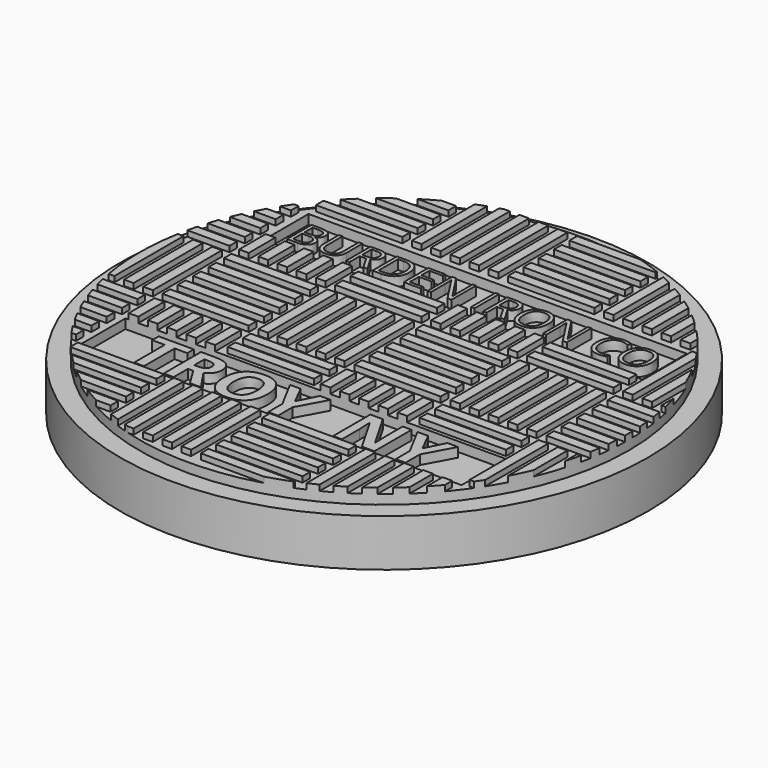
from build123d import *

# Parameters (mm, degrees)
F0_R           = 27.94
F1_DEPTH       = 6
F2_W           = 1.016
F2_H           = 9.144
F2_W_2         = 9.144
F2_H_2         = 1.016
F3_DEPTH       = 0.6
F4_R           = 47.3051944378
F4_R_2         = 27.94
F5_DEPTH       = 25.4
F6_DEPTH       = 5
F7_R           = 27.94
F7_R_2         = 25.908
F8_DEPTH       = 25.4
F9_W           = 40.0505103171
F9_H           = 5.9277797118
F10_DEPTH      = 25.4
F11_TEXT_SIZE  = 4.5379089589
F12_DEPTH      = 1
F12_DEPTH_BACK = 1
F13_W          = 40.3386186808
F13_H          = 5.9581985697
F14_DEPTH      = 25.4
F15_TEXT_SIZE  = 6.8953818821
F16_DEPTH      = 1


# Not quite as in the source:
# - Text() gives the source's letters only with a copy of the font that has no kerning and outlines rounded to 1/6400 em; it was checked with that copy


with BuildPart() as f1:
    # F0 (on Top) → F1 (new body)
    with BuildSketch(Plane.XY):
        Circle(F0_R)
    extrude(amount=F1_DEPTH)

    # F2 (on face) → F3 (join)
    with BuildSketch(Plane.XY.offset(6)):
        with Locations((-9.144, 0)):
            Rectangle(F2_W, F2_H)
        with Locations((-7.112, 0)):
            Rectangle(F2_W, F2_H)
        with Locations((-5.08, 0)):
            Rectangle(F2_W, F2_H)
        with Locations((-3.048, 0)):
            Rectangle(F2_W, F2_H)
        with Locations((-1.016, 0)):
            Rectangle(F2_W, F2_H)
        with Locations((5.08, 4.064)):
            Rectangle(F2_W_2, F2_H_2)
        with Locations((5.08, 2.032)):
            Rectangle(F2_W_2, F2_H_2)
        with Locations((5.08, 0)):
            Rectangle(F2_W_2, F2_H_2)
        with Locations((5.08, -2.032)):
            Rectangle(F2_W_2, F2_H_2)
        with Locations((5.08, -4.064)):
            Rectangle(F2_W_2, F2_H_2)
        with Locations((-5.08, 14.224)):
            Rectangle(F2_W_2, F2_H_2)
        with Locations((-5.08, 12.192)):
            Rectangle(F2_W_2, F2_H_2)
        with Locations((-5.08, 10.16)):
            Rectangle(F2_W_2, F2_H_2)
        with Locations((-5.08, 8.128)):
            Rectangle(F2_W_2, F2_H_2)
        with Locations((-5.08, 6.096)):
            Rectangle(F2_W_2, F2_H_2)
        with Locations((1.016, 10.16)):
            Rectangle(F2_W, F2_H)
        with Locations((3.048, 10.16)):
            Rectangle(F2_W, F2_H)
        with Locations((5.08, 10.16)):
            Rectangle(F2_W, F2_H)
        with Locations((7.112, 10.16)):
            Rectangle(F2_W, F2_H)
        with Locations((9.144, 10.16)):
            Rectangle(F2_W, F2_H)
        with Locations((25.4, -2.032)):
            Rectangle(F2_W_2, F2_H_2)
        with Locations((15.24, 14.224)):
            Rectangle(F2_W_2, F2_H_2)
        with Locations((15.24, 10.16)):
            Rectangle(F2_W_2, F2_H_2)
        with Locations((19.304, 0)):
            Rectangle(F2_W, F2_H)
        with Locations((15.24, 6.096)):
            Rectangle(F2_W_2, F2_H_2)
        with Locations((17.272, 0)):
            Rectangle(F2_W, F2_H)
        with Locations((23.368, 10.16)):
            Rectangle(F2_W, F2_H)
        with Locations((15.24, 12.192)):
            Rectangle(F2_W_2, F2_H_2)
        with Locations((25.4, 10.16)):
            Rectangle(F2_W, F2_H)
        with Locations((21.336, 10.16)):
            Rectangle(F2_W, F2_H)
        with Locations((27.432, 10.16)):
            Rectangle(F2_W, F2_H)
        with Locations((25.4, 2.032)):
            Rectangle(F2_W_2, F2_H_2)
        with Locations((15.24, 8.128)):
            Rectangle(F2_W_2, F2_H_2)
        with Locations((25.4, 0)):
            Rectangle(F2_W_2, F2_H_2)
        with Locations((25.4, -4.064)):
            Rectangle(F2_W_2, F2_H_2)
        with Locations((29.464, 10.16)):
            Rectangle(F2_W, F2_H)
        with Locations((15.24, 0)):
            Rectangle(F2_W, F2_H)
        with Locations((13.208, 0)):
            Rectangle(F2_W, F2_H)
        with Locations((11.176, 0)):
            Rectangle(F2_W, F2_H)
        with Locations((25.4, 4.064)):
            Rectangle(F2_W_2, F2_H_2)
        with Locations((-25.4, 8.128)):
            Rectangle(F2_W_2, F2_H_2)
        with Locations((-15.24, 10.16)):
            Rectangle(F2_W, F2_H)
        with Locations((-15.24, 4.064)):
            Rectangle(F2_W_2, F2_H_2)
        with Locations((-15.24, -4.064)):
            Rectangle(F2_W_2, F2_H_2)
        with Locations((-15.24, 2.032)):
            Rectangle(F2_W_2, F2_H_2)
        with Locations((-25.4, 14.224)):
            Rectangle(F2_W_2, F2_H_2)
        with Locations((-25.4, 6.096)):
            Rectangle(F2_W_2, F2_H_2)
        with Locations((-13.208, 10.16)):
            Rectangle(F2_W, F2_H)
        with Locations((-17.272, 10.16)):
            Rectangle(F2_W, F2_H)
        with Locations((-25.4, 10.16)):
            Rectangle(F2_W_2, F2_H_2)
        with Locations((-21.336, 0)):
            Rectangle(F2_W, F2_H)
        with Locations((-15.24, -2.032)):
            Rectangle(F2_W_2, F2_H_2)
        with Locations((-19.304, 10.16)):
            Rectangle(F2_W, F2_H)
        with Locations((-23.368, 0)):
            Rectangle(F2_W, F2_H)
        with Locations((-25.4, 0)):
            Rectangle(F2_W, F2_H)
        with Locations((-11.176, 10.16)):
            Rectangle(F2_W, F2_H)
        with Locations((-27.432, 0)):
            Rectangle(F2_W, F2_H)
        with Locations((-29.464, 0)):
            Rectangle(F2_W, F2_H)
        with Locations((-25.4, 12.192)):
            Rectangle(F2_W_2, F2_H_2)
        with Locations((-15.24, 0)):
            Rectangle(F2_W_2, F2_H_2)
        with Locations((15.24, 28.448)):
            Rectangle(F2_W_2, F2_H_2)
        with Locations((15.24, 34.544)):
            Rectangle(F2_W_2, F2_H_2)
        with Locations((3.048, 30.48)):
            Rectangle(F2_W, F2_H)
        with Locations((25.4, 20.32)):
            Rectangle(F2_W_2, F2_H_2)
        with Locations((-15.24, 30.48)):
            Rectangle(F2_W, F2_H)
        with Locations((-15.24, 18.288)):
            Rectangle(F2_W_2, F2_H_2)
        with Locations((-1.016, 20.32)):
            Rectangle(F2_W, F2_H)
        with Locations((-3.048, 20.32)):
            Rectangle(F2_W, F2_H)
        with Locations((11.176, 20.32)):
            Rectangle(F2_W, F2_H)
        with Locations((-23.368, 20.32)):
            Rectangle(F2_W, F2_H)
        with Locations((-5.08, 20.32)):
            Rectangle(F2_W, F2_H)
        with Locations((-7.112, 20.32)):
            Rectangle(F2_W, F2_H)
        with Locations((-25.4, 30.48)):
            Rectangle(F2_W_2, F2_H_2)
        with Locations((-9.144, 20.32)):
            Rectangle(F2_W, F2_H)
        with Locations((15.24, 32.512)):
            Rectangle(F2_W_2, F2_H_2)
        with Locations((15.24, 30.48)):
            Rectangle(F2_W_2, F2_H_2)
        with Locations((5.08, 18.288)):
            Rectangle(F2_W_2, F2_H_2)
        with Locations((25.4, 22.352)):
            Rectangle(F2_W_2, F2_H_2)
        with Locations((25.4, 16.256)):
            Rectangle(F2_W_2, F2_H_2)
        with Locations((-15.24, 20.32)):
            Rectangle(F2_W_2, F2_H_2)
        with Locations((-5.08, 30.48)):
            Rectangle(F2_W_2, F2_H_2)
        with Locations((-15.24, 22.352)):
            Rectangle(F2_W_2, F2_H_2)
        with Locations((-11.176, 30.48)):
            Rectangle(F2_W, F2_H)
        with Locations((-19.304, 30.48)):
            Rectangle(F2_W, F2_H)
        with Locations((23.368, 30.48)):
            Rectangle(F2_W, F2_H)
        with Locations((15.24, 20.32)):
            Rectangle(F2_W, F2_H)
        with Locations((5.08, 16.256)):
            Rectangle(F2_W_2, F2_H_2)
        with Locations((5.08, 24.384)):
            Rectangle(F2_W_2, F2_H_2)
        with Locations((17.272, 20.32)):
            Rectangle(F2_W, F2_H)
        with Locations((19.304, 20.32)):
            Rectangle(F2_W, F2_H)
        with Locations((5.08, 30.48)):
            Rectangle(F2_W, F2_H)
        with Locations((-5.08, 28.448)):
            Rectangle(F2_W_2, F2_H_2)
        with Locations((-25.4, 28.448)):
            Rectangle(F2_W_2, F2_H_2)
        with Locations((27.432, 30.48)):
            Rectangle(F2_W, F2_H)
        with Locations((-25.4, 26.416)):
            Rectangle(F2_W_2, F2_H_2)
        with Locations((-25.4, 20.32)):
            Rectangle(F2_W, F2_H)
        with Locations((21.336, 30.48)):
            Rectangle(F2_W, F2_H)
        with Locations((-25.4, 32.512)):
            Rectangle(F2_W_2, F2_H_2)
        with Locations((-17.272, 30.48)):
            Rectangle(F2_W, F2_H)
        with Locations((7.112, 30.48)):
            Rectangle(F2_W, F2_H)
        with Locations((-25.4, 34.544)):
            Rectangle(F2_W_2, F2_H_2)
        with Locations((25.4, 30.48)):
            Rectangle(F2_W, F2_H)
        with Locations((-15.24, 24.384)):
            Rectangle(F2_W_2, F2_H_2)
        with Locations((5.08, 22.352)):
            Rectangle(F2_W_2, F2_H_2)
        with Locations((-5.08, 34.544)):
            Rectangle(F2_W_2, F2_H_2)
        with Locations((-5.08, 26.416)):
            Rectangle(F2_W_2, F2_H_2)
        with Locations((15.24, 26.416)):
            Rectangle(F2_W_2, F2_H_2)
        with Locations((29.464, 30.48)):
            Rectangle(F2_W, F2_H)
        with Locations((25.4, 24.384)):
            Rectangle(F2_W_2, F2_H_2)
        with Locations((5.08, 20.32)):
            Rectangle(F2_W_2, F2_H_2)
        with Locations((25.4, 18.288)):
            Rectangle(F2_W_2, F2_H_2)
        with Locations((9.144, 30.48)):
            Rectangle(F2_W, F2_H)
        with Locations((-5.08, 32.512)):
            Rectangle(F2_W_2, F2_H_2)
        with Locations((-27.432, 20.32)):
            Rectangle(F2_W, F2_H)
        with Locations((-21.336, 20.32)):
            Rectangle(F2_W, F2_H)
        with Locations((13.208, 20.32)):
            Rectangle(F2_W, F2_H)
        with Locations((1.016, 30.48)):
            Rectangle(F2_W, F2_H)
        with Locations((-29.464, 20.32)):
            Rectangle(F2_W, F2_H)
        with Locations((-13.208, 30.48)):
            Rectangle(F2_W, F2_H)
        with Locations((-15.24, 16.256)):
            Rectangle(F2_W_2, F2_H_2)
        with Locations((-15.24, -22.352)):
            Rectangle(F2_W_2, F2_H_2)
        with Locations((-15.24, -10.16)):
            Rectangle(F2_W, F2_H)
        with Locations((17.272, -20.32)):
            Rectangle(F2_W, F2_H)
        with Locations((19.304, -20.32)):
            Rectangle(F2_W, F2_H)
        with Locations((25.4, -20.32)):
            Rectangle(F2_W_2, F2_H_2)
        with Locations((3.048, -10.16)):
            Rectangle(F2_W, F2_H)
        with Locations((15.24, -6.096)):
            Rectangle(F2_W_2, F2_H_2)
        with Locations((-21.336, -20.32)):
            Rectangle(F2_W, F2_H)
        with Locations((15.24, -12.192)):
            Rectangle(F2_W_2, F2_H_2)
        with Locations((-25.4, -8.128)):
            Rectangle(F2_W_2, F2_H_2)
        with Locations((-5.08, -10.16)):
            Rectangle(F2_W_2, F2_H_2)
        with Locations((25.4, -18.288)):
            Rectangle(F2_W_2, F2_H_2)
        with Locations((5.08, -22.352)):
            Rectangle(F2_W_2, F2_H_2)
        with Locations((5.08, -20.32)):
            Rectangle(F2_W_2, F2_H_2)
        with Locations((5.08, -10.16)):
            Rectangle(F2_W, F2_H)
        with Locations((25.4, -22.352)):
            Rectangle(F2_W_2, F2_H_2)
        with Locations((9.144, -10.16)):
            Rectangle(F2_W, F2_H)
        with Locations((-5.08, -8.128)):
            Rectangle(F2_W_2, F2_H_2)
        with Locations((15.24, -20.32)):
            Rectangle(F2_W, F2_H)
        with Locations((-27.432, -20.32)):
            Rectangle(F2_W, F2_H)
        with Locations((-25.4, -6.096)):
            Rectangle(F2_W_2, F2_H_2)
        with Locations((-25.4, -10.16)):
            Rectangle(F2_W_2, F2_H_2)
        with Locations((-23.368, -20.32)):
            Rectangle(F2_W, F2_H)
        with Locations((11.176, -20.32)):
            Rectangle(F2_W, F2_H)
        with Locations((15.24, -14.224)):
            Rectangle(F2_W_2, F2_H_2)
        with Locations((13.208, -20.32)):
            Rectangle(F2_W, F2_H)
        with Locations((-25.4, -14.224)):
            Rectangle(F2_W_2, F2_H_2)
        with Locations((-1.016, -20.32)):
            Rectangle(F2_W, F2_H)
        with Locations((27.432, -10.16)):
            Rectangle(F2_W, F2_H)
        with Locations((1.016, -10.16)):
            Rectangle(F2_W, F2_H)
        with Locations((29.464, -10.16)):
            Rectangle(F2_W, F2_H)
        with Locations((-17.272, -10.16)):
            Rectangle(F2_W, F2_H)
        with Locations((-15.24, -20.32)):
            Rectangle(F2_W_2, F2_H_2)
        with Locations((25.4, -24.384)):
            Rectangle(F2_W_2, F2_H_2)
        with Locations((15.24, -10.16)):
            Rectangle(F2_W_2, F2_H_2)
        with Locations((15.24, -8.128)):
            Rectangle(F2_W_2, F2_H_2)
        with Locations((25.4, -10.16)):
            Rectangle(F2_W, F2_H)
        with Locations((-13.208, -10.16)):
            Rectangle(F2_W, F2_H)
        with Locations((-29.464, -20.32)):
            Rectangle(F2_W, F2_H)
        with Locations((5.08, -16.256)):
            Rectangle(F2_W_2, F2_H_2)
        with Locations((5.08, -24.384)):
            Rectangle(F2_W_2, F2_H_2)
        with Locations((-5.08, -12.192)):
            Rectangle(F2_W_2, F2_H_2)
        with Locations((-25.4, -12.192)):
            Rectangle(F2_W_2, F2_H_2)
        with Locations((-11.176, -10.16)):
            Rectangle(F2_W, F2_H)
        with Locations((21.336, -10.16)):
            Rectangle(F2_W, F2_H)
        with Locations((-15.24, -16.256)):
            Rectangle(F2_W_2, F2_H_2)
        with Locations((25.4, -16.256)):
            Rectangle(F2_W_2, F2_H_2)
        with Locations((23.368, -10.16)):
            Rectangle(F2_W, F2_H)
        with Locations((-19.304, -10.16)):
            Rectangle(F2_W, F2_H)
        with Locations((-15.24, -24.384)):
            Rectangle(F2_W_2, F2_H_2)
        with Locations((7.112, -10.16)):
            Rectangle(F2_W, F2_H)
        with Locations((-5.08, -14.224)):
            Rectangle(F2_W_2, F2_H_2)
        with Locations((-5.08, -6.096)):
            Rectangle(F2_W_2, F2_H_2)
        with Locations((5.08, -18.288)):
            Rectangle(F2_W_2, F2_H_2)
        with Locations((-15.24, -18.288)):
            Rectangle(F2_W_2, F2_H_2)
        with Locations((-25.4, -20.32)):
            Rectangle(F2_W, F2_H)
        with Locations((-3.048, -20.32)):
            Rectangle(F2_W, F2_H)
        with Locations((-9.144, -20.32)):
            Rectangle(F2_W, F2_H)
        with Locations((-7.112, -20.32)):
            Rectangle(F2_W, F2_H)
        with Locations((-5.08, -20.32)):
            Rectangle(F2_W, F2_H)
    extrude(amount=F3_DEPTH)

    # F4 (on face) → F5 (cut)
    with BuildSketch(Plane(origin=(0, 0, 0), x_dir=(1, 0, 0), z_dir=(0, 0, -1))):
        Circle(F4_R)
        Circle(F4_R_2, mode=Mode.SUBTRACT)
    extrude(amount=-F5_DEPTH, mode=Mode.SUBTRACT)

    # F7 (on face) → F8 (cut)
    with BuildSketch(Plane.XY.offset(5)):
        Circle(F7_R)
        Circle(F7_R_2, mode=Mode.SUBTRACT)
    extrude(amount=F8_DEPTH, mode=Mode.SUBTRACT)

    # F9 (on face) → F10 (cut)
    with BuildSketch(Plane.XY.offset(5)):
        with Locations((0.0054370612, 12.0622985996)):
            Rectangle(F9_W, F9_H)
    extrude(amount=F10_DEPTH, mode=Mode.SUBTRACT)



with BuildPart() as f6:
    # F0 (on Top) → F6 (new body)
    with BuildSketch(Plane.XY):
        Circle(F0_R)
    extrude(amount=F6_DEPTH)


with BuildPart() as f1_1:
    add(f1.part)

    add(f6.part)  # F12 merges F6
    # F11 (on face) → F12 (join, two sides)
    with BuildSketch(Plane.XY.offset(5)) as f12_sk:
        with Locations((-19.05, 10.414)):
            Text('BURDEN IRON CO', F11_TEXT_SIZE, font='Open Sans', text_align=(TextAlign.LEFT, TextAlign.BOTTOM))
    extrude(amount=F12_DEPTH)
    extrude(f12_sk.sketch, amount=-F12_DEPTH_BACK)

    # F13 (on face) → F14 (cut)
    with BuildSketch(Plane.XY.offset(5)):
        with Locations((0.0129351392, -12.0018939488)):
            Rectangle(F13_W, F13_H)
    extrude(amount=F14_DEPTH, mode=Mode.SUBTRACT)

    # F15 (on face) → F16 (join)
    with BuildSketch(Plane.XY.offset(5)):
        with Locations((-16.1378871128, -14.7436749551)):
            Text('TROY  NY', F15_TEXT_SIZE, font='Open Sans', font_style=FontStyle.BOLD, text_align=(TextAlign.LEFT, TextAlign.BOTTOM))
    extrude(amount=F16_DEPTH)


solid = f1_1.part
